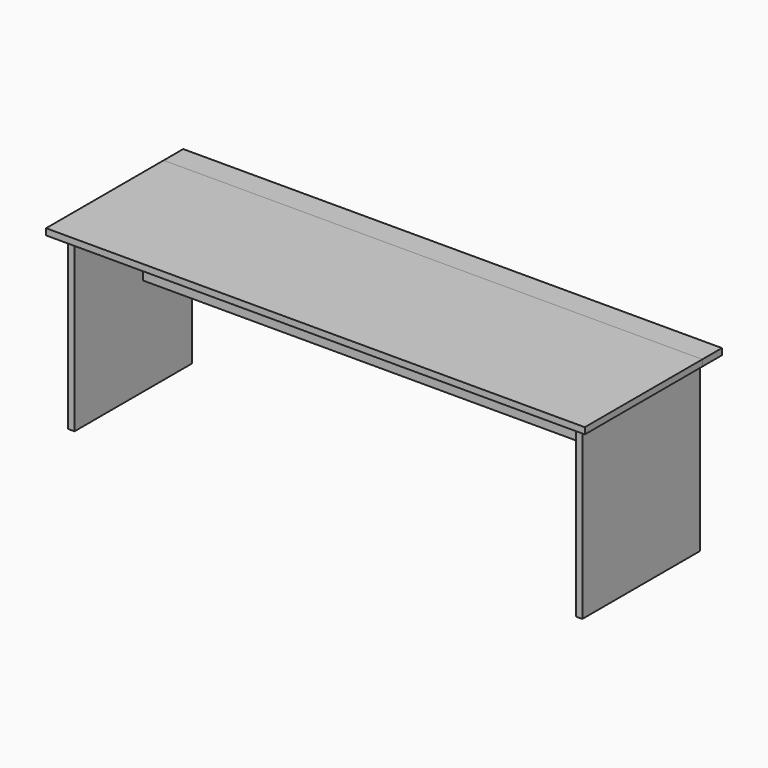
from build123d import *

# Parameters (mm, degrees)
F0_W     = 2200
F0_H     = 600
F1_DEPTH = 26
F0_H_2   = 100
F2_DEPTH = 26
F3_W     = 26
F3_H     = 50
F4_DEPTH = 700
F3_W_2   = 2048
F3_H_2   = 26
F5_DEPTH = 300


# Not quite as in the source:
# - a feature of the source that left no trace in its solid (it failed there, or was rolled back) is left out


with BuildPart() as f1:
    # F0 (on Top) → F1 (new body)
    with BuildSketch(Plane.XY):
        with Locations((1100, 300)):
            Rectangle(F0_W, F0_H)
    extrude(amount=-F1_DEPTH)


with BuildPart() as f2:
    # F0 (on Top) → F2 (new body)
    with BuildSketch(Plane.XY):
        with Locations((1100, 650)):
            Rectangle(F0_W, F0_H_2)
    extrude(amount=-F2_DEPTH)


with BuildPart() as f4:
    # F3 (on face) → F4 (new body)
    with BuildSketch(Plane(origin=(0, 0, -26), x_dir=(1, 0, 0), z_dir=(0, 0, -1))):
        Polygon((2124, -426), (2124, -600), (2150, -600), (2150, -50), (2124, -50), (2124, -400), align=None)
        with Locations((2137, -625)):
            Rectangle(F3_W, F3_H)
    extrude(amount=F4_DEPTH)


with BuildPart() as f4b:
    # F3 (on face) → F4, piece 2 (new body)
    with BuildSketch(Plane(origin=(0, 0, -26), x_dir=(1, 0, 0), z_dir=(0, 0, -1))):
        Polygon((50, -600), (76, -600), (76, -426), (76, -400), (76, -50), (50, -50), align=None)
        with Locations((63, -625)):
            Rectangle(F3_W, F3_H)
    extrude(amount=F4_DEPTH)


with BuildPart() as f5:
    # F3 (on face) → F5 (new body)
    with BuildSketch(Plane(origin=(0, 0, -26), x_dir=(1, 0, 0), z_dir=(0, 0, -1))):
        with Locations((1100, -413)):
            Rectangle(F3_W_2, F3_H_2)
    extrude(amount=F5_DEPTH)


solid = Compound([f1.part, f2.part, f4.part, f4b.part, f5.part])
